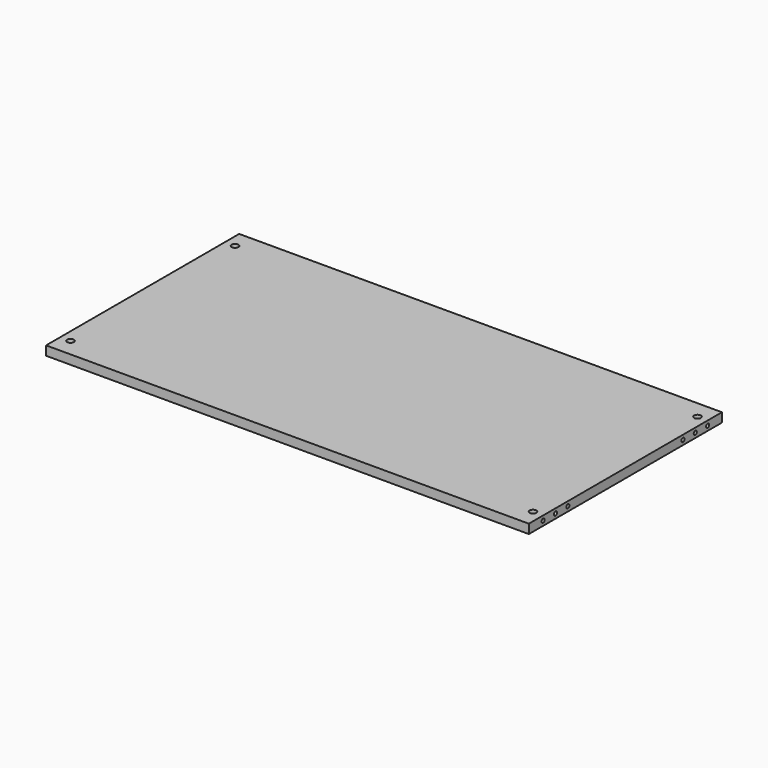
from build123d import *

# Parameters (mm, degrees)
F0_W             = 1000
F0_H             = 500
F1_DEPTH         = 19
F2_R             = 7
F3_DEPTH         = 14
F4_R             = 4
F5_DEPTH         = 25
F5_COPIES2_COUNT = 2


# Not quite as in the source:
# - a pattern or mirror of a feature is missing from the dataset's text; its kind, count and spacing are read off the source's solid


with BuildPart() as f1:
    # F0 (on Top) → F1 (new body)
    with BuildSketch(Plane.XY):
        Rectangle(F0_W, F0_H)
    extrude(amount=F1_DEPTH)

    # F2 (on face) → F3 (cut)
    with BuildSketch(Plane.XY.offset(19)):
        with Locations((-479, -213)):
            Circle(F2_R)
    f3 = extrude(amount=-F3_DEPTH, mode=Mode.SUBTRACT)

    # F3_copies: F3 across plane
    add(f3.mirror(Plane(origin=(0, 0, 0), x_dir=(-0.4063154508, 0.9137328682, 0), z_dir=(0.9137328682, 0.4063154508, 0))), mode=Mode.SUBTRACT)

    # F3_copies1: F3 across plane
    add(f3.mirror(Plane(origin=(0, 0, 0), x_dir=(0, 0, 1), z_dir=(1, 0, 0))), mode=Mode.SUBTRACT)

    # F3_copies2: F3 across plane
    add(f3.mirror(Plane.ZX), mode=Mode.SUBTRACT)

    # F4 (on face) → F5 (cut)
    with BuildSketch(Plane(origin=(-500, 0, 0), x_dir=(0, -1, 0), z_dir=(-1, 0, 0))):
        with Locations((213, 9.5)):
            Circle(F4_R)
        with Locations((181, 9.5)):
            Circle(F4_R)
        with Locations((149, 9.5)):
            Circle(F4_R)
    f5 = extrude(amount=-F5_DEPTH, mode=Mode.SUBTRACT)

    # F5_copies: F5 across plane
    add(f5.mirror(Plane(origin=(0, 0, 0), x_dir=(0, 0, 1), z_dir=(1, 0, 0))), mode=Mode.SUBTRACT)

    # F5_copies1: F5 across plane
    add(f5.mirror(Plane.ZX), mode=Mode.SUBTRACT)

    # F5_copies2: F5 ×2 about axis
    f5_copies2_axis = Axis((0, 0, 0), (0, 0, 1))
    for i in range(1, F5_COPIES2_COUNT):
        add(f5.rotate(f5_copies2_axis, i * 360 / F5_COPIES2_COUNT), mode=Mode.SUBTRACT)


solid = f1.part
